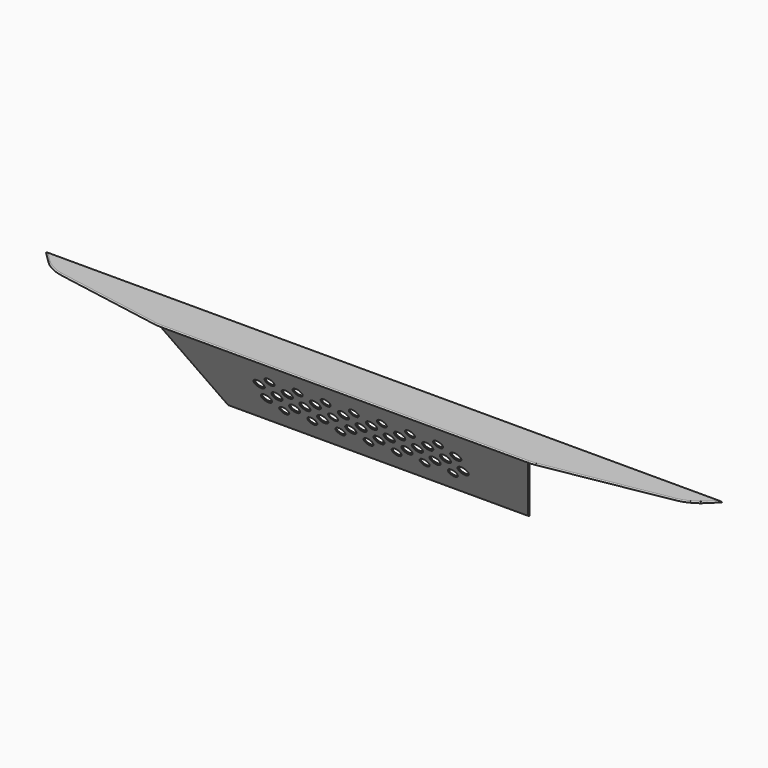
from build123d import *

# Parameters (mm, degrees)
F9_R      = 12.7
F10_DEPTH = 3.175
F11_SIZE  = 1.524
F12_DEPTH = 3.175
F13_R     = 3.17499
F14_DEPTH = 3.175


# Not quite as in the source:
# - a fillet or chamfer is up to 0.001 mm smaller than in the source, because OpenCascade refuses the exact size


with BuildPart() as f10:
    # F9 (on 3pt) → F10 (new body)
    with BuildSketch(Plane(origin=(0, 0, 0), x_dir=(-1, 0, 0), z_dir=(0, 0.8715755371, 0.4902612396))):
        Polygon((-406.0266635338, 0), (406.7733364662, 0), (498.000045759, 233.1410088337), (-498.000045759, 233.1410088337), align=None)
        with Locations((-266.5133317669, 91.1705044169)):
            Circle(F9_R, mode=Mode.SUBTRACT)
        with Locations((-228.4133317669, 65.7705044169)):
            Circle(F9_R, mode=Mode.SUBTRACT)
        with Locations((-152.2133317669, 65.7705044169)):
            Circle(F9_R, mode=Mode.SUBTRACT)
        with Locations((-76.0133317669, 65.7705044169)):
            Circle(F9_R, mode=Mode.SUBTRACT)
        with Locations((-190.3133317669, 91.1705044169)):
            Circle(F9_R, mode=Mode.SUBTRACT)
        with Locations((-114.1133317669, 91.1705044169)):
            Circle(F9_R, mode=Mode.SUBTRACT)
        with Locations((-37.9133317669, 91.1705044169)):
            Circle(F9_R, mode=Mode.SUBTRACT)
        with Locations((0.1866682331, 65.7705044169)):
            Circle(F9_R, mode=Mode.SUBTRACT)
        with Locations((76.3866682331, 65.7705044169)):
            Circle(F9_R, mode=Mode.SUBTRACT)
        with Locations((152.5866682331, 65.7705044169)):
            Circle(F9_R, mode=Mode.SUBTRACT)
        with Locations((228.7866682331, 65.7705044169)):
            Circle(F9_R, mode=Mode.SUBTRACT)
        with Locations((38.2866682331, 91.1705044169)):
            Circle(F9_R, mode=Mode.SUBTRACT)
        with Locations((114.4866682331, 91.1705044169)):
            Circle(F9_R, mode=Mode.SUBTRACT)
        with Locations((190.6866682331, 91.1705044169)):
            Circle(F9_R, mode=Mode.SUBTRACT)
        with Locations((266.8866682331, 91.1705044169)):
            Circle(F9_R, mode=Mode.SUBTRACT)
        with Locations((-266.5133317669, 141.9705044169)):
            Circle(F9_R, mode=Mode.SUBTRACT)
        with Locations((-228.4133317669, 116.5705044169)):
            Circle(F9_R, mode=Mode.SUBTRACT)
        with Locations((-152.2133317669, 116.5705044169)):
            Circle(F9_R, mode=Mode.SUBTRACT)
        with Locations((-190.3133317669, 141.9705044169)):
            Circle(F9_R, mode=Mode.SUBTRACT)
        with Locations((-76.0133317669, 116.5705044169)):
            Circle(F9_R, mode=Mode.SUBTRACT)
        with Locations((-114.1133317669, 141.9705044169)):
            Circle(F9_R, mode=Mode.SUBTRACT)
        with Locations((-37.9133317669, 141.9705044169)):
            Circle(F9_R, mode=Mode.SUBTRACT)
        with Locations((-228.4133317669, 167.3705044169)):
            Circle(F9_R, mode=Mode.SUBTRACT)
        with Locations((-152.2133317669, 167.3705044169)):
            Circle(F9_R, mode=Mode.SUBTRACT)
        with Locations((-76.0133317669, 167.3705044169)):
            Circle(F9_R, mode=Mode.SUBTRACT)
        with Locations((0.1866682331, 116.5705044169)):
            Circle(F9_R, mode=Mode.SUBTRACT)
        with Locations((76.3866682331, 116.5705044169)):
            Circle(F9_R, mode=Mode.SUBTRACT)
        with Locations((38.2866682331, 141.9705044169)):
            Circle(F9_R, mode=Mode.SUBTRACT)
        with Locations((114.4866682331, 141.9705044169)):
            Circle(F9_R, mode=Mode.SUBTRACT)
        with Locations((152.5866682331, 116.5705044169)):
            Circle(F9_R, mode=Mode.SUBTRACT)
        with Locations((228.7866682331, 116.5705044169)):
            Circle(F9_R, mode=Mode.SUBTRACT)
        with Locations((190.6866682331, 141.9705044169)):
            Circle(F9_R, mode=Mode.SUBTRACT)
        with Locations((0.1866682331, 167.3705044169)):
            Circle(F9_R, mode=Mode.SUBTRACT)
        with Locations((76.3866682331, 167.3705044169)):
            Circle(F9_R, mode=Mode.SUBTRACT)
        with Locations((152.5866682331, 167.3705044169)):
            Circle(F9_R, mode=Mode.SUBTRACT)
        with Locations((228.7866682331, 167.3705044169)):
            Circle(F9_R, mode=Mode.SUBTRACT)
        with Locations((266.8866682331, 141.9705044169)):
            Circle(F9_R, mode=Mode.SUBTRACT)
    extrude(amount=F10_DEPTH)

    # F11
    f11_edges = [f10.edges().sort_by_distance(p)[0] for p in [
        (126.813332, -44.697365, 79.461981),
        (-254.186668, -69.602635, 123.738019),
        (-177.986668, -69.602635, 123.738019),
        (-216.086668, -57.15, 101.6),
        (-254.186668, -44.697365, 79.461981),
        (-177.986668, -44.697365, 79.461981),
        (-139.886668, -57.15, 101.6),
        (-101.786668, -69.602635, 123.738019),
        (-101.786668, -44.697365, 79.461981),
        (-63.686668, -54.382748, 103.156579),
        (-25.586668, -69.602635, 123.738019),
        (-25.586668, -44.697365, 79.461981),
        (12.513332, -57.15, 101.6),
        (50.613332, -69.602635, 123.738019),
        (50.613332, -44.697365, 79.461981),
        (88.713332, -57.15, 101.6),
        (126.813332, -69.602635, 123.738019),
        (164.913332, -57.15, 101.6),
        (203.013332, -69.602635, 123.738019),
        (279.213332, -69.602635, 123.738019),
        (241.113332, -57.15, 101.6),
        (203.013332, -44.697365, 79.461981),
        (279.213332, -44.697365, 79.461981),
    ]]
    chamfer(f11_edges, length=F11_SIZE)

    # F2 (on offset) → F12 (join)
    with BuildSketch(Plane.XY.offset(203.2)):
        with BuildLine():
            Line((-498.000045759, -114.3), (498.000045759, -114.3))
            ThreePointArc((498.000045759, -114.3), (507.961947155, -113.8650539919), (517.8480324663, -112.5635261693))
            Line((517.8480324663, -112.5635261693), (849.2502458829, -54.1283744775))
            ThreePointArc((849.2502458829, -54.1283744775), (882.1801256683, -42.9501865404), (910.2245642651, -22.3871533978))
            Line((910.2245642651, -22.3871533978), (932.6117176629, 0))
            Line((932.6117176629, 0), (-900.5608627483, 0))
            Line((-900.5608627483, 0), (-871.3124545275, -29.2484082208))
            ThreePointArc((-871.3124545275, -29.2484082208), (-843.2680159306, -49.8114413635), (-810.3381361452, -60.9896293005))
            Line((-810.3381361452, -60.9896293005), (-517.8480324663, -112.5635261693))
            ThreePointArc((-517.8480324663, -112.5635261693), (-507.961947155, -113.8650539919), (-498.000045759, -114.3))
        make_face()
    extrude(amount=F12_DEPTH)

    # F13 (radius 3.175 in the source; OpenCascade refuses exactly that, so slightly less here)
    f13_edges = [f10.edges().sort_by_distance(p)[0] for p in [
        (-843.268016, -49.811441, 206.375),
        (-664.093084, -86.776578, 206.375),
        (-507.961947, -113.865054, 206.375),
        (0, -114.3, 206.375),
        (507.961947, -113.865054, 206.375),
        (683.549139, -83.34595, 206.375),
        (882.180126, -42.950187, 206.375),
        (921.418141, -11.193577, 206.375),
        (16.025427, 0, 206.375),
        (-885.936659, -14.624204, 206.375),
    ]]
    fillet(f13_edges, radius=F13_R)

    # F6 (on 3pt) + F4 (on 3pt) → F14 (join)
    with BuildSketch(Plane(origin=(246.4519411848, 198.3116236809, 0), x_dir=(-0.6269093852, 0.7790921786, 0), z_dir=(0.7790921786, 0.6269093852, 0))):
        Polygon((-254.5419260156, 203.2), (-401.2511385345, 203.2), (-254.5419260156, 0), align=None)
    with BuildSketch(Plane(origin=(-248.484372052, 198.3238107874, 0), x_dir=(0.6238053284, 0.7815797543, 0), z_dir=(0.7815797543, -0.6238053284, 0))):
        Polygon((-253.7473747264, 203.2), (-399.9896479869, 203.2), (-253.7473747264, 0), align=None)
    extrude(amount=F14_DEPTH, dir=(0.7790921786, 0.6269093852, 0))


solid = f10.part
